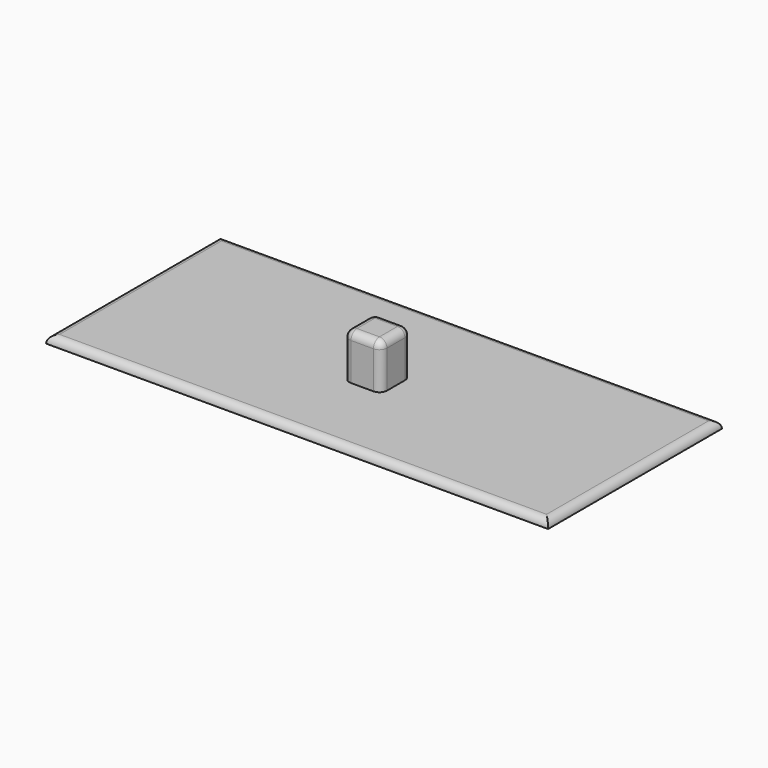
from build123d import *

# Parameters (mm, degrees)
F0_W     = 170.18
F0_H     = 73.66
F1_DEPTH = 2.54
F2_W     = 12.7
F2_H     = 12.7
F3_DEPTH = 15.24
F4_R     = 2.53999


# Not quite as in the source:
# - a fillet or chamfer is up to 0.001 mm smaller than in the source, because OpenCascade refuses the exact size


with BuildPart() as f1:
    # F0 (on Top) → F1 (new body)
    with BuildSketch(Plane.XY):
        with Locations((1.0795005364, 0)):
            Rectangle(F0_W, F0_H)
    extrude(amount=F1_DEPTH)

    # F2 (on face) → F3 (join)
    with BuildSketch(Plane.XY.offset(2.54)):
        with Locations((0, -1.5238544315)):
            Rectangle(F2_W, F2_H)
    extrude(amount=F3_DEPTH)

    # F4 (radius 2.54 in the source; OpenCascade refuses exactly that, so slightly less here)
    f4_edges = [f1.edges().sort_by_distance(p)[0] for p in [
        (0, -7.873854, 17.78),
        (-6.35, -1.523854, 17.78),
        (0, 4.826146, 17.78),
        (6.35, -1.523854, 17.78),
        (-6.35, -7.873854, 10.16),
        (6.35, -7.873854, 10.16),
        (6.35, 4.826146, 10.16),
        (-6.35, 4.826146, 10.16),
        (1.079501, -36.83, 2.54),
        (86.169501, 0, 2.54),
        (1.079501, 36.83, 2.54),
        (-84.010499, 0, 2.54),
    ]]
    fillet(f4_edges, radius=F4_R)


solid = f1.part
